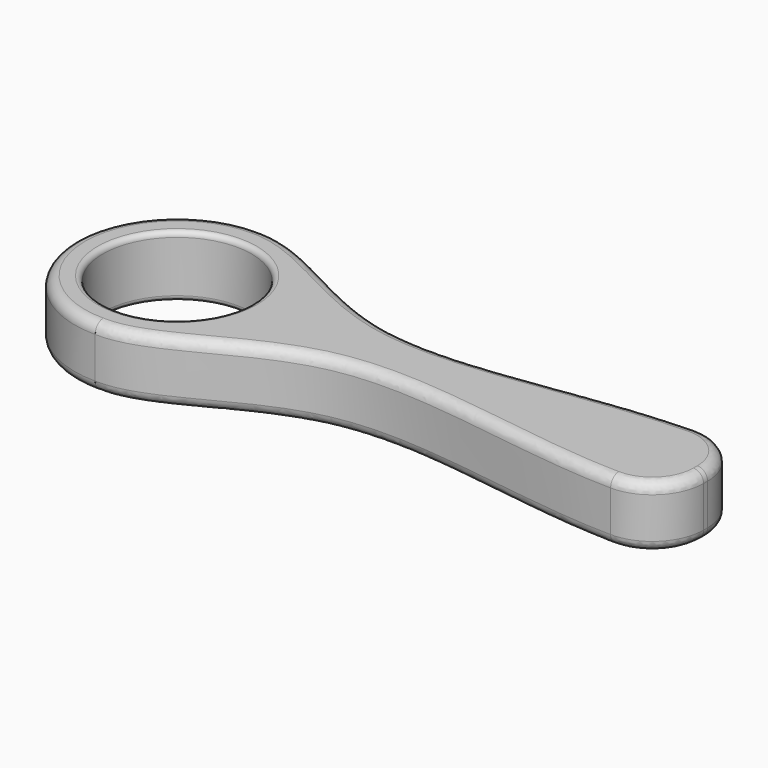
from build123d import *

# Parameters (mm, degrees)
F0_R     = 7.25
F1_DEPTH = 6
F2_R     = 5
F3_R     = 1
F4_R     = 0.5
F5_R     = 0.5


# Not quite as in the source:
# - a feature names something its author has since deleted; it is built from what else it names


with BuildPart() as f1:
    # F0 (on Top) → F1 (new body)
    with BuildSketch(Plane.XY):
        with BuildLine():
            ThreePointArc((0, -10), (7.0710678119, -7.0710678119), (10, 0))
            ThreePointArc((10, 0), (7.0710678119, 7.0710678119), (0, 10))
            ThreePointArc((0, 10), (-10, 0), (0, -10))
        make_face()
        Circle(F0_R, mode=Mode.SUBTRACT)
        with BuildLine():
            ThreePointArc((0, 10), (7.0710678119, 7.0710678119), (10, 0))
            ThreePointArc((10, 0), (7.0710678119, -7.0710678119), (0, -10))
            add(Edge.make_bspline(
                [(0, -10), (5.1704310233, -10.1955717475), (17.8057120766, 2.2538375417), (39.9110362514, -6.3769862775), (51.5451952815, -5)],
                knots=[0, 0, 0, 0, 0.4275250723, 1, 1, 1, 1], degree=3))
            Line((51.5451952815, -5), (51.5451952815, 5))
            add(Edge.make_bspline(
                [(0, 10), (5.1704310233, 10.1955717475), (17.8057120766, -2.2538375417), (39.9110362514, 6.3769862775), (51.5451952815, 5)],
                knots=[0, 0, 0, 0, 0.4275250723, 1, 1, 1, 1], degree=3))
        make_face()
    extrude(amount=F1_DEPTH)

    # F2
    f2_edges = [f1.edges().sort_by_distance(p)[0] for p in [
        (51.545195, -5, 3),
        (51.545195, 5, 3),
    ]]
    fillet(f2_edges, radius=F2_R)

    # F3
    f3_edges = [f1.edges().sort_by_distance(p)[0] for p in [
        (-10, 0, 6),
        (-10, 0, 0),
        (19.299517, -3.140676, 0),
        (19.299517, -3.140676, 6),
        (50.055771, -3.802235, 0),
        (51.545195, 0, 0),
        (19.299517, 3.140676, 0),
        (50.055771, 3.802235, 0),
        (50.055771, -3.802235, 6),
        (51.545195, 0, 6),
        (19.299517, 3.140676, 6),
        (50.055771, 3.802235, 6),
    ]]
    fillet(f3_edges, radius=F3_R)

    # F4
    f4_edges = [f1.edges().sort_by_distance(p)[0] for p in [
        (-7.25, 0, 0),
    ]]
    fillet(f4_edges, radius=F4_R)

    # F5
    f5_edges = [f1.edges().sort_by_distance(p)[0] for p in [
        (-7.25, 0, 6),
    ]]
    fillet(f5_edges, radius=F5_R)


solid = f1.part
